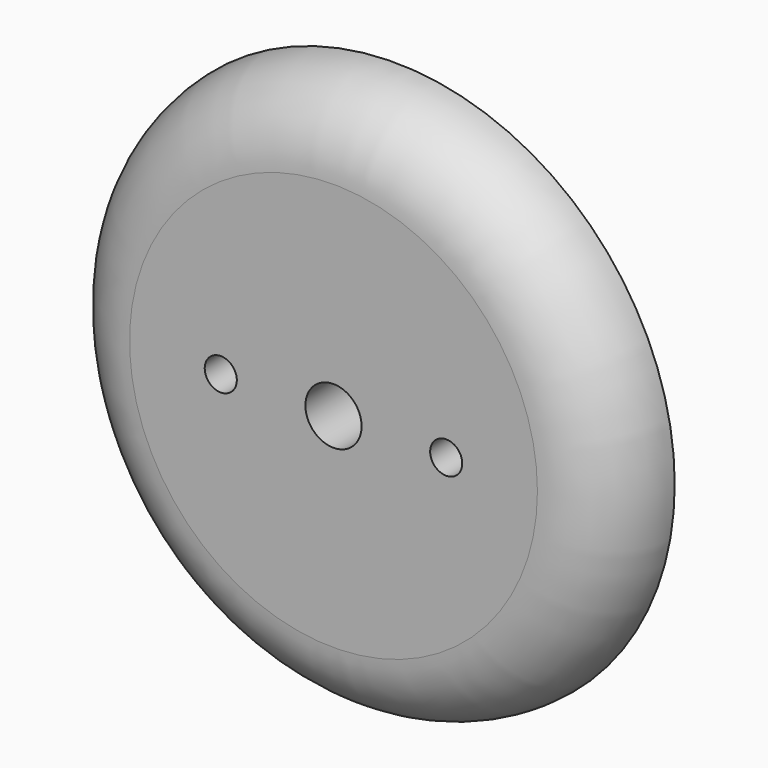
from build123d import *

# Parameters (mm, degrees)
F0_R           = 69.8
F0_R_2         = 5
F1_DEPTH       = 19
F2_R           = 18.99999
F3_D           = 14
F3_DEPTH       = 20
F3_TIP         = 4.2060243332
F4_D           = 8
F4_DEPTH       = 20
F4_CSINK_D     = 25
F4_CSINK_ANGLE = 100
F4_TIP         = 2.4034424761


# Not quite as in the source:
# - a fillet or chamfer is up to 0.001 mm smaller than in the source, because OpenCascade refuses the exact size


with BuildPart() as f1:
    # F0 (on Front) → F1 (new body)
    with BuildSketch(Plane.XZ):
        Circle(F0_R)
        with Locations((-28.077211231, 0)):
            Circle(F0_R_2, mode=Mode.SUBTRACT)
        with Locations((28.077211231, 0)):
            Circle(F0_R_2, mode=Mode.SUBTRACT)
        with Locations((-28.077211231, 0)):
            Circle(F0_R_2)
        with Locations((28.077211231, 0)):
            Circle(F0_R_2)
    extrude(amount=F1_DEPTH)

    # F2 (radius 19 in the source; OpenCascade refuses exactly that, so slightly less here)
    f2_edges = [f1.edges().sort_by_distance(p)[0] for p in [
        (-69.8, -19, 0),
    ]]
    fillet(f2_edges, radius=F2_R)

    # F3
    with Locations(Plane(origin=(0, 0, 0), x_dir=(1, 0, 0), z_dir=(0, 1, 0))):
        with Locations((0, 0)):
            Hole(F3_D / 2, depth=F3_DEPTH)
            with Locations((0, 0, -(F3_DEPTH + F3_TIP / 2))):  # 118° drill point
                Cone(0, F3_D / 2, F3_TIP, mode=Mode.SUBTRACT)

    # F4
    with Locations(Plane(origin=(0, 0, 0), x_dir=(1, 0, 0), z_dir=(0, 1, 0))):
        with Locations((28.077211231, 0), (-28.077211231, 0)):
            CounterSinkHole(F4_D / 2, F4_CSINK_D / 2, depth=F4_DEPTH, counter_sink_angle=F4_CSINK_ANGLE)
            with Locations((0, 0, -(F4_DEPTH + F4_TIP / 2))):  # 118° drill point
                Cone(0, F4_D / 2, F4_TIP, mode=Mode.SUBTRACT)


solid = f1.part
